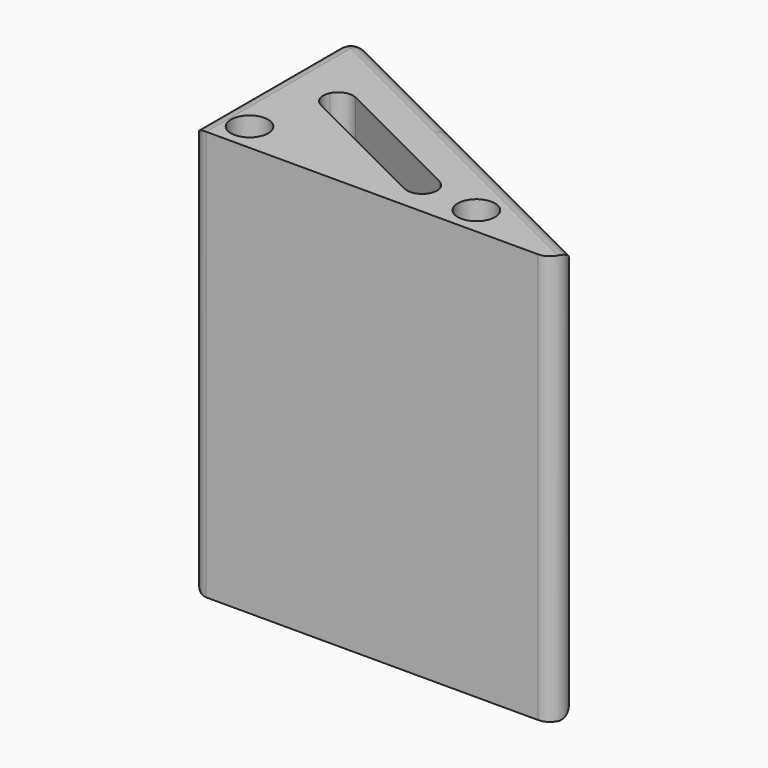
from build123d import *

# Parameters (mm, degrees)
F0_R     = 1
F1_DEPTH = 22
F3_R     = 0.79999


# Not quite as in the source:
# - a fillet or chamfer is up to 0.001 mm smaller than in the source, because OpenCascade refuses the exact size
# - a feature of the source that left no trace in its solid (it failed there, or was rolled back) is left out


with BuildPart() as f1:
    # F0 (on Top) → F1 (new body)
    with BuildSketch(Plane.XY):
        Polygon((0, 10), (0, 0), (20, 0), (22, 0), (8.6841676623, 6.6579161689), (0, 11), align=None)
        with Locations((1.9193962216, 1.5117339551)):
            Circle(F0_R, mode=Mode.SUBTRACT)
        Polygon((3.0234679102, 6.6994116629), (9.2844582472, 3.5689164944), (11.9677398202, 2.2272757079), (11.6099689438, 1.5117339551), (11.2521980674, 0.7961922023), (9.8211145618, 1.5117339551), (7.0483902697, 2.8980961012), (4.3426890694, 4.2509467013), (2.3079261574, 5.2683281573), align=None, mode=Mode.SUBTRACT)
        with BuildLine():
            ThreePointArc((15.0937268734, 1.5117339551), (14.0937268734, 0.5117339551), (13.0937268734, 1.5117339551))
            ThreePointArc((13.0937268734, 1.5117339551), (14.0937268734, 2.5117339551), (15.0937268734, 1.5117339551))
        make_face(mode=Mode.SUBTRACT)
    extrude(amount=F1_DEPTH)

    # F3 (radius 0.8 in the source; OpenCascade refuses exactly that, so slightly less here)
    f3_edges = [f1.edges().sort_by_distance(p)[0] for p in [
        (0, 11, 11),
        (22, 0, 11),
        (11, 5.5, 0),
        (11, 5.5, 22),
        (0, 5.5, 22),
        (2.307926, 5.268328, 11),
        (3.023468, 6.699412, 11),
        (11.252198, 0.796192, 11),
        (11.96774, 2.227276, 11),
        (0, 0, 11),
        (0, 5.5, 0),
    ]]
    fillet(f3_edges, radius=F3_R)


solid = f1.part
